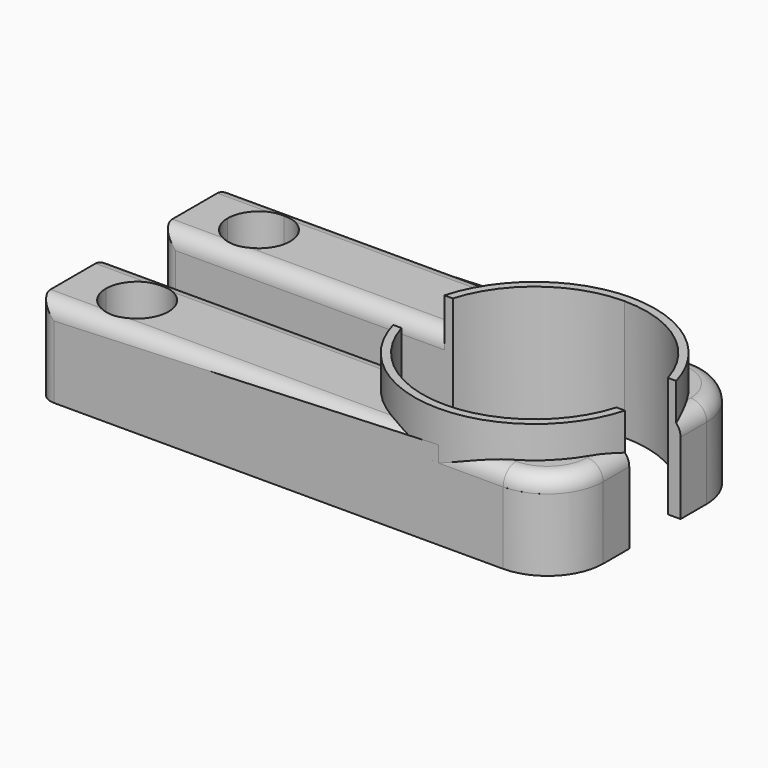
from build123d import *
from build123d import SkipClean  # not in build123d's __all__

# Parameters (mm, degrees)
F1_DEPTH     = 11
F2_DEPTH     = 15
F4_T1_DEPTH  = 21
F4_T6_DEPTH  = 63.5
F4_S7_R      = 15
F4_T8_DEPTH  = 33
F4_T12_DEPTH = 45.5431677052
F4_S13_R     = 15
F4_T14_DEPTH = 24
F5_DEPTH     = 11
F6_R         = 2
F7_T1_DEPTH  = 28.5024142421
F7_T4_ANGLE  = 90


# Not quite as in the source:
# - a fillet or chamfer that OpenCascade refuses, or shapes differently, is made with other operations: its cross-section is extruded or revolved along the edge and cut away or added


with BuildPart() as f1:
    # F0 (on Top) → F1 (new body)
    with BuildSketch(Plane.XY):
        with BuildLine():
            Line((8, 0), (0, 0))
            Line((0, 0), (0, -5.5))
            Line((0, -5.5), (4.1, -5.5))
            ThreePointArc((4.1, -5.5), (5.2422835534, -2.7422835534), (8, -1.6))
            Line((8, -1.6), (8, 0))
        make_face()
        with BuildLine():
            Line((50, 0), (8, 0))
            Line((8, 0), (8, -1.6))
            ThreePointArc((8, -1.6), (10.7577164466, -2.7422835534), (11.9, -5.5))
            ThreePointArc((11.9, -5.5), (8, -9.4), (4.1, -5.5))
            Line((4.1, -5.5), (0, -5.5))
            Line((0, -5.5), (0, -11))
            Line((0, -11), (35.5431677052, -11))
            ThreePointArc((35.5431677052, -11), (40.9170489377, -3.0626636137), (50, 0))
        make_face()
    extrude(amount=F1_DEPTH)

    # F0 (on Top) → F2 (join)
    with BuildSketch(Plane.XY):
        with BuildLine():
            Line((50, -1), (50, 0))
            ThreePointArc((50, 0), (40.9170489377, -3.0626636137), (35.5431677052, -11))
            Line((35.5431677052, -11), (36.583592135, -11))
            ThreePointArc((36.583592135, -11), (41.6333997347, -3.7750278397), (50, -1))
        make_face()
        with BuildLine():
            ThreePointArc((64.4568322948, -11), (59.0829510623, -3.0626636137), (50, 0))
            Line((50, 0), (50, -1))
            ThreePointArc((50, -1), (58.3666002653, -3.7750278397), (63.416407865, -11))
            Line((63.416407865, -11), (64.4568322948, -11))
        make_face()
    extrude(amount=F2_DEPTH)

    # F4: fillet of radius 2 on 4 edges, made by hand

    # F4_s2 → F4_t1 (cut)
    with BuildSketch(Plane.XY.offset(-5)):
        with BuildLine():
            ThreePointArc((0, -2), (0.5857864376, -0.5857864376), (2, 0))
            Line((2, 0), (0, 0))
            Line((0, 0), (0, -2))
        make_face()
        with BuildLine():
            ThreePointArc((0, -9), (0.5857864376, -10.4142135624), (2, -11))
            Line((2, -11), (0, -11))
            Line((0, -11), (0, -9))
        make_face()
    extrude(amount=F4_T1_DEPTH, mode=Mode.SUBTRACT)


with BuildPart() as f4_tool4:
    # F4_s5 → F4_t6 (new body)
    with BuildSketch(Plane.YZ.offset(58.5)):
        with BuildLine():
            ThreePointArc((-2, 11), (-0.5857864376, 10.4142135624), (0, 9))
            Line((0, 9), (0, 11))
            Line((0, 11), (-2, 11))
        make_face()
    extrude(amount=-F4_T6_DEPTH)

    # F4_s7 → F4_t8 (cut, symmetric)
    with BuildSketch(Plane.XY.offset(10)):
        with Locations((50, -15)):
            Circle(F4_S7_R)
    extrude(amount=F4_T8_DEPTH, both=True, mode=Mode.SUBTRACT)


with BuildPart() as f1_1:
    add(f1.part, clean=False)

    # F4_t3: cut F4_tool4
    add(f4_tool4.part, mode=Mode.SUBTRACT)


with BuildPart() as f4_tool10:
    # F4_s11 → F4_t12 (new body)
    with BuildSketch(Plane.YZ.offset(-5)):
        with BuildLine():
            ThreePointArc((-9, 11), (-10.4142135624, 10.4142135624), (-11, 9))
            Line((-11, 9), (-11, 11))
            Line((-11, 11), (-9, 11))
        make_face()
    extrude(amount=F4_T12_DEPTH)

    # F4_s13 → F4_t14 (cut, symmetric)
    with BuildSketch(Plane.XY.offset(10)):
        with Locations((50, -15)):
            Circle(F4_S13_R)
    extrude(amount=F4_T14_DEPTH, both=True, mode=Mode.SUBTRACT)


with BuildPart() as f1_2:
    add(f1_1.part, clean=False)

    # F4_t9: cut F4_tool10
    add(f4_tool10.part, mode=Mode.SUBTRACT)

    # F0 (on Top) → F5 (join)
    with BuildSketch(Plane.XY):
        with BuildLine():
            Line((65, 0), (50, 0))
            ThreePointArc((50, 0), (59.0829510623, -3.0626636137), (64.4568322948, -11))
            Line((64.4568322948, -11), (65, -11))
            Line((65, -11), (65, 0))
        make_face()
    extrude(amount=F5_DEPTH)

    # F6
    f6_edges = [f1_2.edges().sort_by_distance(p)[0] for p in [
        (57.5, 0, 11),
        (65, -5.5, 11),
    ]]
    fillet(f6_edges, radius=F6_R)

    # F7: fillet of radius 7 on 1 edges, made by hand

    # F7_s2 → F7_t1 (cut)
    with BuildSketch(Plane.XY.offset(-17.5024142421)):
        with BuildLine():
            ThreePointArc((65.0004, -7.0009656854), (62.9497474683, -2.0502525317), (57.9990343146, 0.0004))
            Line((57.9990343146, 0.0004), (57.9990343146, 0.7005365685))
            ThreePointArc((57.9990343146, 0.7005365685), (61.4995171573, 0.7001365685), (65, 0.7001365685))
            Line((65, 0.7001365685), (65.7001365685, 0))
            ThreePointArc((65.7001365685, 0), (65.7001365685, -3.5004828427), (65.7005365685, -7.0009656854))
            Line((65.7005365685, -7.0009656854), (65.0004, -7.0009656854))
        make_face()
    with SkipClean():  # cleaning this boolean's faces spoils the solid; the shape is the same uncleaned
        extrude(amount=F7_T1_DEPTH, mode=Mode.SUBTRACT)

    # F7_s3 → F7_t4 (revolve, cut)
    with BuildSketch(Plane.XZ.offset(7.0009656854)):
        with BuildLine():
            ThreePointArc((63.0004, 11), (64.4146135624, 10.4142135624), (65.0004, 9))
            Line((65.0004, 9), (65.0004, 11))
            Line((65.0004, 11), (63.0004, 11))
        make_face()
    with SkipClean():  # cleaning this boolean's faces spoils the solid; the shape is the same uncleaned
        revolve(axis=Axis((57.9990343146, -7.0009656854, 11), (0, 0, 1)), revolution_arc=F7_T4_ANGLE, mode=Mode.SUBTRACT)


with BuildPart() as f8_1:
    # F8: instance of F1
    add(f1_2.part.mirror(Plane.XZ.offset(15)), clean=False)


solid = Compound([f1_2.part, f8_1.part])
